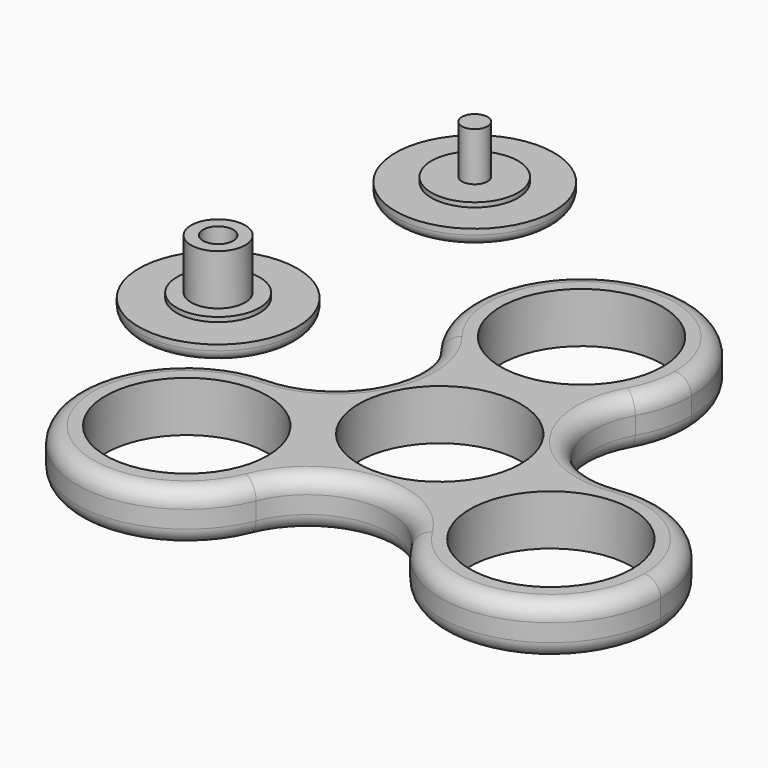
from build123d import *

# Parameters (mm, degrees)
F0_R      = 11.25
F1_DEPTH  = 7
F2_R      = 2.286
F3_R      = 2.286
F4_R      = 11
F4_R_2    = 5.75
F5_DEPTH  = 1.27
F4_R_3    = 3.75
F6_DEPTH  = 1.905
F4_R_4    = 2.0955
F7_DEPTH  = 8.905
F8_R      = 11
F8_R_2    = 6
F9_DEPTH  = 1.27
F8_R_3    = 1.778
F10_DEPTH = 1.905
F11_DEPTH = 8.65
F12_DEPTH = 1
F13_R     = 9.3604062529
F13_R_2   = 1.778
F14_DEPTH = 1
F16_R     = 1.5
F17_DEPTH = 1
F18_R     = 9.360408
F19_DEPTH = 1
F21_R     = 1.5


# Not quite as in the source:
# - a fillet or chamfer that OpenCascade refuses, or shapes differently, is made with other operations: its cross-section is extruded or revolved along the edge and cut away or added


with BuildPart() as f1:
    # F0 (on Top) → F1 (new body)
    with BuildSketch(Plane.XY):
        with BuildLine():
            ThreePointArc((-8.4611516462, -21.3015945231), (-7.6457254486, -18.5219963455), (-7.3706078777, -15.6383534697))
            ThreePointArc((-7.3706078777, -15.6383534697), (-11.9425890824, -4.7506349481), (-22.9171540556, -0.3912370091))
            ThreePointArc((-22.9171540556, -0.3912370091), (-35.1647631553, -24.310531303), (-8.4611516462, -21.3015945231))
        make_face()
        with Locations((-22.6206078777, -15.6383534697)):
            Circle(F0_R, mode=Mode.SUBTRACT)
        with BuildLine():
            ThreePointArc((-22.9171540556, -0.3912370091), (-11.9425890824, -4.7506349481), (-7.3706078777, -15.6383534697))
            ThreePointArc((-7.3706078777, -15.6383534697), (-7.6457254486, -18.5219963455), (-8.4611516462, -21.3015945231))
            ThreePointArc((-8.4611516462, -21.3015945231), (1.1570520367, -14.202947954), (11.7973982166, -19.6512190901))
            ThreePointArc((11.7973982166, -19.6512190901), (11.0711113685, -5.2433761134), (22.6782978212, 3.3232249907))
            ThreePointArc((22.6782978212, 3.3232249907), (11.7215877184, 8.1035104343), (11.119755839, 20.0424560992))
            ThreePointArc((11.119755839, 20.0424560992), (-0.9946587684, 12.2095517499), (-14.217146175, 17.9783695324))
            ThreePointArc((-14.217146175, 17.9783695324), (-12.8786397552, 6.0994375197), (-22.9171540556, -0.3912370091))
        make_face()
        Circle(F0_R, mode=Mode.SUBTRACT)
        with BuildLine():
            ThreePointArc((13.0170925607, 27.409197806), (-7.223040668, 41.8196478461), (-14.217146175, 17.9783695324))
            ThreePointArc((-14.217146175, 17.9783695324), (-0.9946587684, 12.2095517499), (11.119755839, 20.0424560992))
            ThreePointArc((11.119755839, 20.0424560992), (12.5351427873, 23.605621528), (13.0170925607, 27.409197806))
        make_face()
        with Locations((-2.2329074393, 27.409197806)):
            Circle(F0_R, mode=Mode.SUBTRACT)
        with BuildLine():
            ThreePointArc((22.6782978212, 3.3232249907), (11.0711113685, -5.2433761134), (11.7973982166, -19.6512190901))
            ThreePointArc((11.7973982166, -19.6512190901), (28.9435467483, -26.4621391359), (40.103515317, -11.7708443362))
            ThreePointArc((40.103515317, -11.7708443362), (34.8382645174, -0.2440371718), (22.6782978212, 3.3232249907))
        make_face()
        with Locations((24.853515317, -11.7708443362)):
            Circle(F0_R, mode=Mode.SUBTRACT)
    extrude(amount=F1_DEPTH)

    # F2
    f2_edges = [f1.edges().sort_by_distance(p)[0] for p in [
        (-35.164763, -24.310531, 7),
    ]]
    fillet(f2_edges, radius=F2_R)

    # F3
    f3_edges = [f1.edges().sort_by_distance(p)[0] for p in [
        (-3.471156, 42.608844, 0),
        (-35.164763, -24.310531, 0),
        (-12.87864, 6.099438, 0),
        (1.157052, -14.202948, 0),
        (38.635919, -18.298313, 0),
        (11.721588, 8.10351, 0),
    ]]
    fillet(f3_edges, radius=F3_R)


with BuildPart() as f5:
    # F4 (on Top) → F5 (new body)
    with BuildSketch(Plane.XY):
        with Locations((-45.6172116101, 18.5634717345)):
            Circle(F4_R)
        with Locations((-45.6172116101, 18.5634717345)):
            Circle(F4_R_2, mode=Mode.SUBTRACT)
    extrude(amount=F5_DEPTH)

    # F4 (on Top) → F6 (join)
    with BuildSketch(Plane.XY):
        with Locations((-45.6172116101, 18.5634717345)):
            Circle(F4_R_2)
        with Locations((-45.6172116101, 18.5634717345)):
            Circle(F4_R_3, mode=Mode.SUBTRACT)
    extrude(amount=F6_DEPTH)



with BuildPart() as f6:
    # F4 (on Top) → F6, piece 2 (new body)
    with BuildSketch(Plane.XY):
        with Locations((-45.6172116101, 18.5634717345)):
            Circle(F4_R_4)
    extrude(amount=F6_DEPTH)


with BuildPart() as f5_1:
    add(f5.part)

    add(f6.part)  # F7 merges F6
    # F4 (on Top) → F7 (join)
    with BuildSketch(Plane.XY):
        with Locations((-45.6172116101, 18.5634717345)):
            Circle(F4_R_3)
        with Locations((-45.6172116101, 18.5634717345)):
            Circle(F4_R_4, mode=Mode.SUBTRACT)
    extrude(amount=F7_DEPTH)

    # F4 (on Top) → F17 (join)
    with BuildSketch(Plane.XY):
        with Locations((-45.6172116101, 18.5634717345)):
            Circle(F4_R)
        with Locations((-45.6172116101, 18.5634717345)):
            Circle(F4_R_2, mode=Mode.SUBTRACT)
        with Locations((-45.6172116101, 18.5634717345)):
            Circle(F4_R_2)
        with Locations((-45.6172116101, 18.5634717345)):
            Circle(F4_R_3, mode=Mode.SUBTRACT)
        with Locations((-45.6172116101, 18.5634717345)):
            Circle(F4_R_3)
        with Locations((-45.6172116101, 18.5634717345)):
            Circle(F4_R_4, mode=Mode.SUBTRACT)
        with Locations((-45.6172116101, 18.5634717345)):
            Circle(F4_R_4)
    extrude(amount=-F17_DEPTH)

    # F18 (on face) → F19 (cut)
    with BuildSketch(Plane(origin=(0, 0, -1), x_dir=(1, 0, 0), z_dir=(0, 0, -1))):
        with Locations((-45.6172116101, -18.5634717345)):
            Circle(F18_R)
    extrude(amount=-F19_DEPTH, mode=Mode.SUBTRACT)

    # F20: fillet of radius 5.08 on 1 edges, made by hand

    # F20_s1 → F20_t2 (revolve)
    with BuildSketch(Plane.XZ.offset(-18.5634717345)):
        with BuildLine():
            ThreePointArc((-36.2568036101, -1), (-37.6896150551, -0.2564743185), (-39.2833528002, 0))
            Line((-39.2833528002, 0), (-36.2568036101, 0))
            Line((-36.2568036101, 0), (-36.2568036101, -1))
        make_face()
    revolve(axis=Axis((-45.6172116101, 18.5634717345, 0), (0, 0, -1)))

    # F21
    f21_edges = [f5_1.edges().sort_by_distance(p)[0] for p in [
        (-56.617212, 18.563472, -1),
    ]]
    fillet(f21_edges, radius=F21_R)


with BuildPart() as f9:
    # F8 (on Top) → F9 (new body)
    with BuildSketch(Plane.XY):
        with Locations((-40.870603174, 57.1643747389)):
            Circle(F8_R)
        with Locations((-40.870603174, 57.1643747389)):
            Circle(F8_R_2, mode=Mode.SUBTRACT)
    extrude(amount=F9_DEPTH)

    # F8 (on Top) → F10 (join)
    with BuildSketch(Plane.XY):
        with Locations((-40.870603174, 57.1643747389)):
            Circle(F8_R_2)
        with Locations((-40.870603174, 57.1643747389)):
            Circle(F8_R_3, mode=Mode.SUBTRACT)
    extrude(amount=F10_DEPTH)

    # F8 (on Top) → F11 (join)
    with BuildSketch(Plane.XY):
        with Locations((-40.870603174, 57.1643747389)):
            Circle(F8_R_3)
    extrude(amount=F11_DEPTH)

    # F8 (on Top) → F12 (join)
    with BuildSketch(Plane.XY):
        with Locations((-40.870603174, 57.1643747389)):
            Circle(F8_R)
        with Locations((-40.870603174, 57.1643747389)):
            Circle(F8_R_2, mode=Mode.SUBTRACT)
        with Locations((-40.870603174, 57.1643747389)):
            Circle(F8_R_2)
        with Locations((-40.870603174, 57.1643747389)):
            Circle(F8_R_3, mode=Mode.SUBTRACT)
    extrude(amount=-F12_DEPTH)

    # F13 (on face) → F14 (cut)
    with BuildSketch(Plane(origin=(0, 0, -1), x_dir=(1, 0, 0), z_dir=(0, 0, -1))):
        with Locations((-40.870603174, -57.1643747389)):
            Circle(F13_R)
        with Locations((-40.870603174, -57.1643747389)):
            Circle(F13_R_2, mode=Mode.SUBTRACT)
    extrude(amount=-F14_DEPTH, mode=Mode.SUBTRACT)

    # F15: fillet of radius 5.08 on 1 edges, made by hand

    # F15_s1 → F15_t2 (revolve)
    with BuildSketch(Plane.XZ.offset(-57.1643747389)):
        with BuildLine():
            ThreePointArc((-31.510196921, -1), (-32.9430083661, -0.2564743185), (-34.5367461111, 0))
            Line((-34.5367461111, 0), (-31.510196921, 0))
            Line((-31.510196921, 0), (-31.510196921, -1))
        make_face()
    revolve(axis=Axis((-40.870603174, 57.1643747389, 0), (0, 0, -1)))

    # F16
    f16_edges = [f9.edges().sort_by_distance(p)[0] for p in [
        (-51.870603, 57.164375, -1),
    ]]
    fillet(f16_edges, radius=F16_R)


solid = Compound([f1.part, f5_1.part, f9.part])
